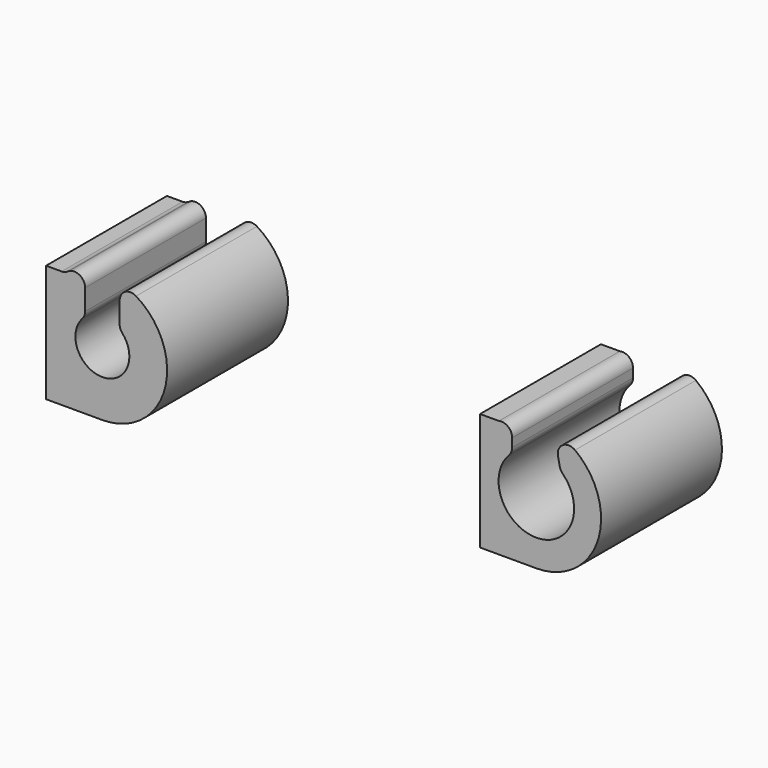
from build123d import *

# Parameters (mm, degrees)
F1_DEPTH    = 7
F2_R        = 0.5
F2_2_R      = 0.5
F3_T1_DEPTH = 11.1105344099


# Not quite as in the source:
# - a fillet or chamfer that OpenCascade refuses, or shapes differently, is made with other operations: its cross-section is extruded or revolved along the edge and cut away or added


with BuildPart() as f1:
    # F0 (on Front) → F1 (new body)
    with BuildSketch(Plane.XZ):
        with BuildLine():
            Line((-0.8, 0.9604686356), (-0.8, 2.891366459))
            ThreePointArc((-0.8, 2.891366459), (-1.2865824769, 2.7101117191), (-1.734622404, 2.4476693232))
            Line((-1.734622404, 2.4476693232), (-2.6087118245, 2.4476693232))
            Line((-2.6087118245, 2.4476693232), (-2.6087118245, 1.4814258728))
            Line((-2.6087118245, 1.4814258728), (-2.6087118245, -1.4814258728))
            Line((-2.6087118245, -1.4814258728), (-2.6087118245, -3))
            Line((-2.6087118245, -3), (0, -3))
            ThreePointArc((0, -3), (2.9727175595, -0.4036710437), (0.8, 2.891366459))
            Line((0.8, 2.891366459), (0.8, 0.9604686356))
            ThreePointArc((0.8, 0.9604686356), (0, -1.25), (-0.8, 0.9604686356))
        make_face()
    extrude(amount=F1_DEPTH)

    # F2
    f2_edges = [f1.edges().sort_by_distance(p)[0] for p in [
        (-0.8, -3.5, 2.891366),
        (-0.8, -3.5, 0.960469),
        (0.8, -3.5, 0.960469),
        (0.8, -3.5, 2.891366),
        (-1.734622, -3.5, 2.447669),
    ]]
    fillet(f2_edges, radius=F2_R)


with BuildPart() as f1b:
    # F0 (on Front) → F1, piece 2 (new body)
    with BuildSketch(Plane.XZ):
        with BuildLine():
            Line((18.987874046, 1.8343775348), (18.987874046, 3.2728132508))
            ThreePointArc((18.987874046, 3.2728132508), (18.6707434577, 3.1230948845), (18.373251642, 2.9373907681))
            Line((18.373251642, 2.9373907681), (17.4991622215, 2.9373907681))
            Line((17.4991622215, 2.9373907681), (17.4991622215, 1.9711473178))
            Line((17.4991622215, 1.9711473178), (17.4991622215, -0.9917044279))
            Line((17.4991622215, -0.9917044279), (17.4991622215, -2.5102785551))
            Line((17.4991622215, -2.5102785551), (20.107874046, -2.5102785551))
            ThreePointArc((20.107874046, -2.5102785551), (23.0805916054, 0.0860504012), (20.907874046, 3.3810879039))
            Line((20.907874046, 3.3810879039), (21.227874046, 1.8343775348))
            ThreePointArc((21.227874046, 1.8343775348), (20.107874046, -1.2602785551), (18.987874046, 1.8343775348))
        make_face()
    extrude(amount=F1_DEPTH)

    # F2#2
    f2_2_edges = [f1b.edges().sort_by_distance(p)[0] for p in [
        (18.987874, -3.5, 1.834378),
        (20.907874, -3.5, 3.381088),
        (21.227874, -3.5, 1.834378),
    ]]
    fillet(f2_2_edges, radius=F2_2_R)

    # F3: fillet of radius 0.5 on 1 edges, made by hand

    # F3_s2 → F3_t1 (cut)
    with BuildSketch(Plane.XZ.offset(-2.055267205)):
        with BuildLine():
            ThreePointArc((18.987874046, 2.4507063688), (18.7982679876, 2.8426956557), (18.373251642, 2.9373907681))
            ThreePointArc((18.373251642, 2.9373907681), (18.6707434577, 3.1230948845), (18.987874046, 3.2728132508))
            Line((18.987874046, 3.2728132508), (18.987874046, 2.4507063688))
        make_face()
    extrude(amount=F3_T1_DEPTH, mode=Mode.SUBTRACT)


solid = Compound([f1.part, f1b.part])
